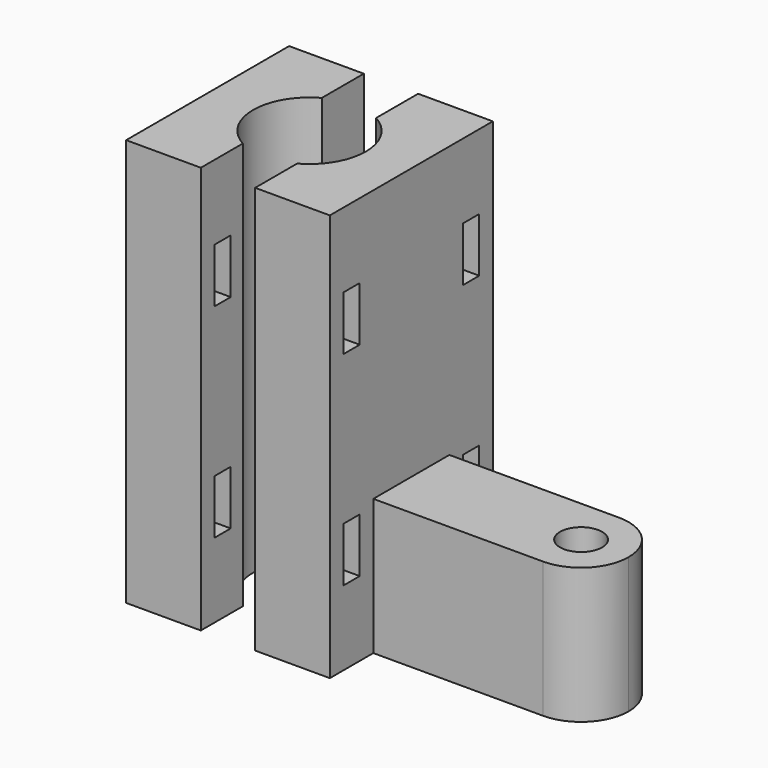
from build123d import *

# Parameters (mm, degrees)
F1_DEPTH = 30
F2_W     = 1.5
F2_H     = 4
F3_DEPTH = 15
F4_DEPTH = 10


# Not quite as in the source:
# - a feature names something its author has since deleted; it is built from what else it names


with BuildPart() as f1:
    # F0 (on Top) → F1 (new body)
    with BuildSketch(Plane.XY):
        with BuildLine():
            ThreePointArc((-2, -3.6362755671), (-4.15, 0), (-2, 3.6362755671))
            Line((-2, 3.6362755671), (-2, 7.5))
            Line((-2, 7.5), (-7.5, 7.5))
            Line((-7.5, 7.5), (-7.5, -7.5))
            Line((-7.5, -7.5), (-2, -7.5))
            Line((-2, -7.5), (-2, -3.6362755671))
        make_face()
    extrude(amount=F1_DEPTH)


with BuildPart() as f1b:
    # F0 (on Top) → F1, piece 2 (new body)
    with BuildSketch(Plane.XY):
        with BuildLine():
            ThreePointArc((2, 3.6362755671), (3.572289182, 2.1121671335), (4.15, 0))
            Line((4.15, 0), (7.5, 0))
            Line((7.5, 0), (7.5, 3.5))
            Line((7.5, 3.5), (7.5, 7.5))
            Line((7.5, 7.5), (2, 7.5))
            Line((2, 7.5), (2, 3.6362755671))
        make_face()
        with BuildLine():
            Line((7.5, 0), (4.15, 0))
            ThreePointArc((4.15, 0), (3.572289182, -2.1121671335), (2, -3.6362755671))
            Line((2, -3.6362755671), (2, -7.5))
            Line((2, -7.5), (7.5, -7.5))
            Line((7.5, -7.5), (7.5, -3.5))
            Line((7.5, -3.5), (7.5, 0))
        make_face()
    extrude(amount=F1_DEPTH)


with BuildPart() as f3_tool:
    # F2 (on face) → F3 (new body, through all)
    with BuildSketch(Plane(origin=(-7.5, 0, 0), x_dir=(0, -1, 0), z_dir=(-1, 0, 0))):
        with Locations((-5.5, 22.5)):
            Rectangle(F2_W, F2_H)
        with Locations((-5.5, 7.5)):
            Rectangle(F2_W, F2_H)
        with Locations((5.5, 7.5)):
            Rectangle(F2_W, F2_H)
        with Locations((5.5, 22.5)):
            Rectangle(F2_W, F2_H)
    extrude(amount=-F3_DEPTH)


with BuildPart() as f1_1:
    add(f1.part)

    # F3: cut by f3_tool
    add(f3_tool.part, mode=Mode.SUBTRACT)


with BuildPart() as f1b_1:
    add(f1b.part)

    # F3: cut by f3_tool
    add(f3_tool.part, mode=Mode.SUBTRACT)

    # F0 (on Top) → F4 (join)
    with BuildSketch(Plane.XY):
        with BuildLine():
            Line((7.5, 3.5), (7.5, 0))
            Line((7.5, 0), (16.5, 0))
            ThreePointArc((16.5, 0), (17.5251262658, 2.4748737342), (20, 3.5))
            Line((20, 3.5), (7.5, 3.5))
        make_face()
        with BuildLine():
            ThreePointArc((20, 3.5), (17.5251262658, 2.4748737342), (16.5, 0))
            ThreePointArc((16.5, 0), (17.5251262658, -2.4748737342), (20, -3.5))
            ThreePointArc((20, -3.5), (22.4748737342, -2.4748737342), (23.5, 0))
            ThreePointArc((23.5, 0), (22.4748737342, 2.4748737342), (20, 3.5))
        make_face()
        with BuildLine():
            ThreePointArc((21.55, 0), (20, -1.55), (18.45, 0))
            ThreePointArc((18.45, 0), (20, 1.55), (21.55, 0))
        make_face(mode=Mode.SUBTRACT)
        with BuildLine():
            Line((16.5, 0), (7.5, 0))
            Line((7.5, 0), (7.5, -3.5))
            Line((7.5, -3.5), (20, -3.5))
            ThreePointArc((20, -3.5), (17.5251262658, -2.4748737342), (16.5, 0))
        make_face()
    extrude(amount=F4_DEPTH)


solid = Compound([f1_1.part, f1b_1.part])
